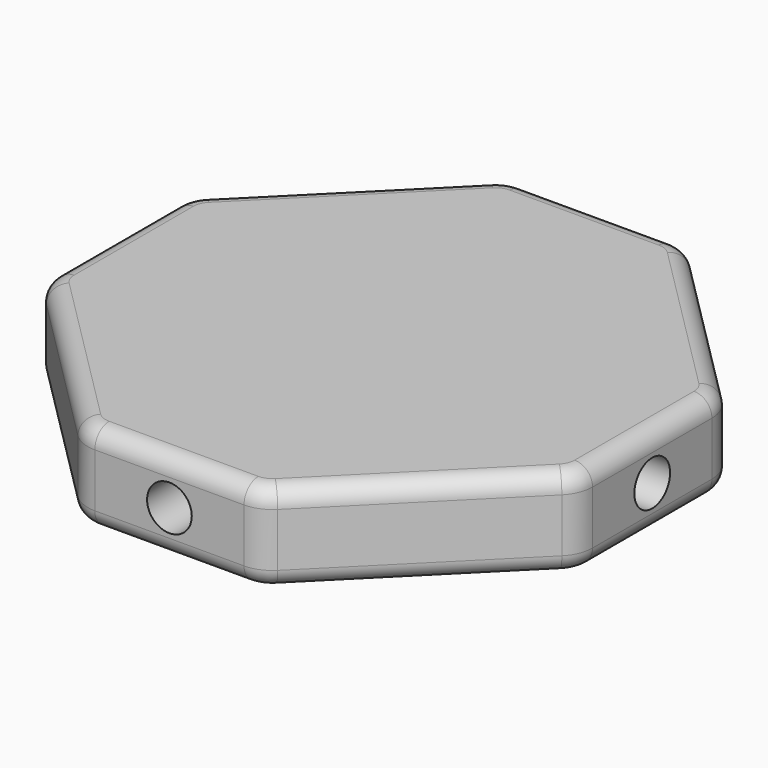
from build123d import *

# Parameters (mm, degrees)
F1_DEPTH = 6.35
F3_D     = 6.35
F4_R     = 5.08
F5_R     = 2.54
F7_D     = 6.35


with BuildPart() as f1:
    # F0 (on Top) → F1 (new body, symmetric)
    with BuildSketch(Plane.XY):
        Polygon((-12.7, 38.1), (-38.1, 12.7), (-38.1, -12.7), (-12.7, -38.1), (12.7, -38.1), (38.1, -12.7), (38.1, 12.7), (12.7, 38.1), align=None)
    extrude(amount=F1_DEPTH, both=True)

    # F3 (through all)
    with Locations(Plane(origin=(-38.1, 0, 0), x_dir=(0, -1, 0), z_dir=(-1, 0, 0))):
        with Locations((0, 0)):
            Hole(F3_D / 2)

    # F4
    f4_edges = [f1.edges().sort_by_distance(p)[0] for p in [
        (-12.7, 38.1, 0),
        (-38.1, 12.7, 0),
        (12.7, 38.1, 0),
        (38.1, 12.7, 0),
        (-38.1, -12.7, 0),
        (-12.7, -38.1, 0),
        (12.7, -38.1, 0),
        (38.1, -12.7, 0),
    ]]
    fillet(f4_edges, radius=F4_R)

    # F5
    f5_edges = [f1.edges().sort_by_distance(p)[0] for p in [
        (-25.4, 25.4, 6.35),
        (-12.539827, 37.713308, 6.35),
        (-37.713308, 12.539827, 6.35),
        (0, 38.1, 6.35),
        (-38.1, 0, 6.35),
        (12.539827, 37.713308, 6.35),
        (-37.713308, -12.539827, 6.35),
        (25.4, 25.4, 6.35),
        (-25.4, -25.4, 6.35),
        (37.713308, 12.539827, 6.35),
        (-12.539827, -37.713308, 6.35),
        (38.1, 0, 6.35),
        (0, -38.1, 6.35),
        (37.713308, -12.539827, 6.35),
        (12.539827, -37.713308, 6.35),
        (25.4, -25.4, 6.35),
        (-25.4, 25.4, -6.35),
        (-12.539827, 37.713308, -6.35),
        (-37.713308, 12.539827, -6.35),
        (0, 38.1, -6.35),
        (-38.1, 0, -6.35),
        (12.539827, 37.713308, -6.35),
        (-37.713308, -12.539827, -6.35),
        (25.4, 25.4, -6.35),
        (-25.4, -25.4, -6.35),
        (37.713308, 12.539827, -6.35),
        (-12.539827, -37.713308, -6.35),
        (38.1, 0, -6.35),
        (0, -38.1, -6.35),
        (37.713308, -12.539827, -6.35),
        (12.539827, -37.713308, -6.35),
        (25.4, -25.4, -6.35),
    ]]
    fillet(f5_edges, radius=F5_R)

    # F7 (through all)
    with Locations(Plane(origin=(0, 38.1, 0), x_dir=(-1, 0, 0), z_dir=(0, 1, 0))):
        with Locations((0, 0)):
            Hole(F7_D / 2)


solid = f1.part
